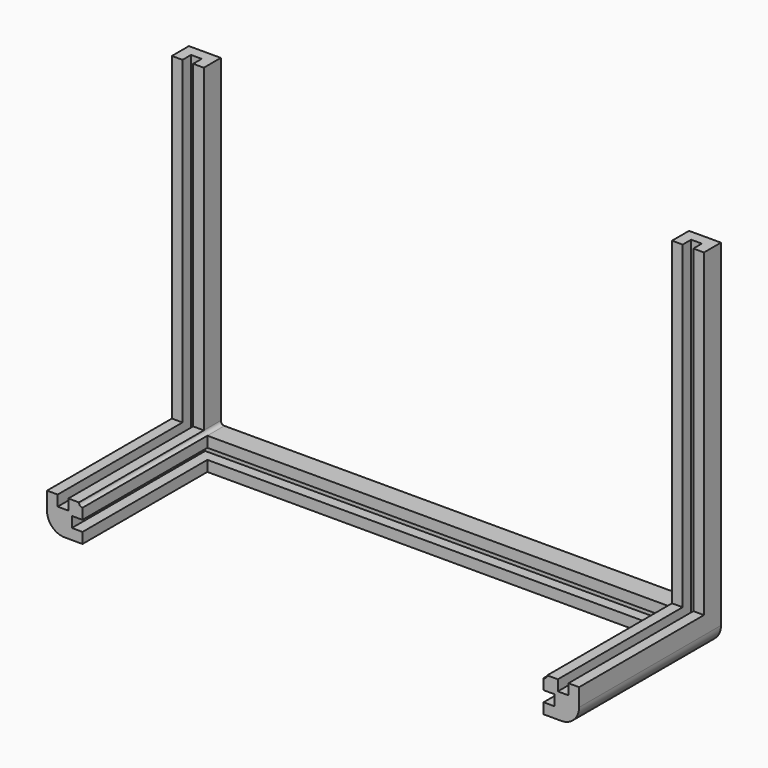
from build123d import *

# Parameters (mm, degrees)
F1_DEPTH = 50
F0_W     = 3
F0_H     = 90
F0_W_2   = 65
F0_H_2   = 3
F2_DEPTH = 6
F3_DEPTH = 3
F4_R     = 0.99999
F5_R     = 5


# Not quite as in the source:
# - a fillet or chamfer is up to 0.001 mm smaller than in the source, because OpenCascade refuses the exact size


with BuildPart() as f1:
    # F0 (on Front) → F1 (new body)
    with BuildSketch(Plane.XZ):
        Polygon((-67, 6), (-65, 6), (-65, 9), (-66, 9), (-66, 10), (-69, 10), (-69, 9), (-69, 7), (-69, 6), (-68, 6), align=None)
        Polygon((-72, 3), (-68, 3), (-68, 6), (-69, 6), (-69, 7), (-72, 7), align=None)
        Polygon((-75, 0), (-65, 0), (-65, 3), (-68, 3), (-72, 3), (-72, 7), (-72, 10), (-75, 10), align=None)
    extrude(amount=F1_DEPTH)

    # F0 (on Front) → F2 (join)
    with BuildSketch(Plane.XZ):
        with Locations((-73.5, 55)):
            Rectangle(F0_W, F0_H)
        with Locations((-67.5, 55)):
            Rectangle(F0_W, F0_H)
        with Locations((-32.5, 7.5)):
            Rectangle(F0_W_2, F0_H_2)
        with Locations((-32.5, 1.5)):
            Rectangle(F0_W_2, F0_H_2)
    extrude(amount=F2_DEPTH)

    # F0 (on Front) → F3 (join)
    with BuildSketch(Plane.XZ):
        Polygon((-72, 100), (-72, 10), (-72, 7), (-69, 7), (-69, 9), (-69, 10), (-69, 100), align=None)
        Polygon((-65, 3), (0, 3), (0, 6), (-65, 6), (-67, 6), (-68, 6), (-68, 3), align=None)
    extrude(amount=F3_DEPTH)

    # F4 (radius 1 in the source; OpenCascade refuses exactly that, so slightly less here)
    f4_edges = [f1.edges().sort_by_distance(p)[0] for p in [
        (-66, -25, 9),
    ]]
    fillet(f4_edges, radius=F4_R)

    # F5
    f5_edges = [f1.edges().sort_by_distance(p)[0] for p in [
        (-75, -25, 0),
    ]]
    fillet(f5_edges, radius=F5_R)

    # F6: F1 across plane


with BuildPart() as f1_1:
    add(f1.part)
    add(f1.part.mirror(Plane.YZ))


solid = f1_1.part
